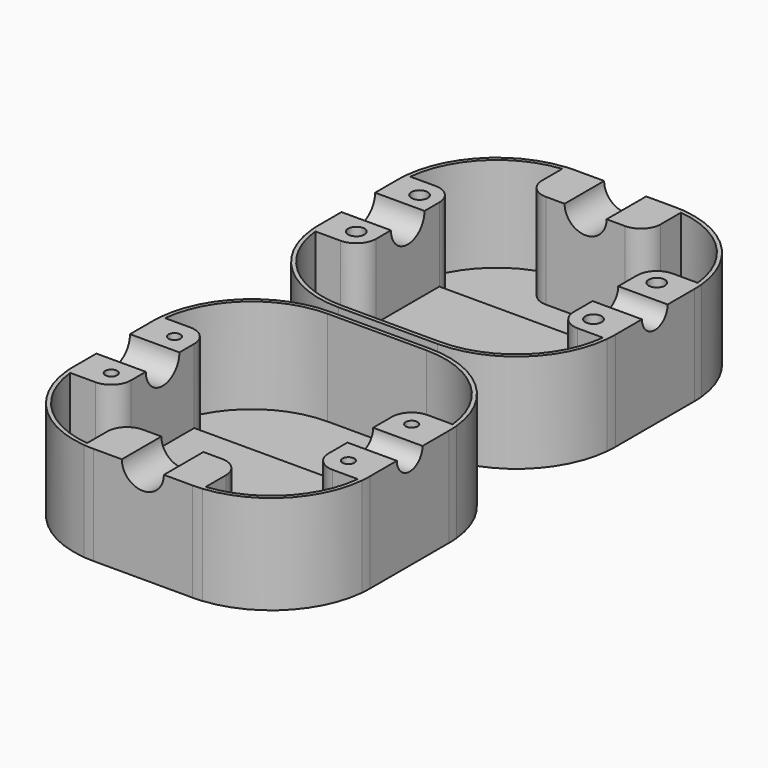
from build123d import *

# Parameters (mm, degrees)
F1_DEPTH        = 20
F2_T            = -0.8
F3_DEPTH        = 5
F4_DEPTH        = 20
F6_D            = 8.5
F6_DEPTH        = 12
F6_TIP          = 2.5536576309
F8_D            = 8.5
F8_DEPTH        = 12
F8_TIP          = 2.5536576309
F10_D           = 6.5
F10_DEPTH       = 12
F10_TIP         = 1.9527970118
F13_D           = 3.3
F13_CBORE_D     = 6.5
F13_CBORE_DEPTH = 6
F15_D           = 2.4
F15_DEPTH       = 17
F15_TIP         = 0.7210327428


# Not quite as in the source:
# - a feature names something its author has since deleted; it is built from what else it names


with BuildPart() as f1:
    # F0 (on Top) → F1 (new body)
    with BuildSketch(Plane.XY):
        with BuildLine():
            Line((-24, -12), (-29.8997487421, -12))
            ThreePointArc((-29.8997487421, -12), (-23.416407865, -24.8323969742), (-10, -30))
            Line((-10, -30), (0, -30))
            Line((0, -30), (10, -30))
            ThreePointArc((10, -30), (23.416407865, -24.8323969742), (29.8997487421, -12))
            Line((29.8997487421, -12), (24, -12))
            ThreePointArc((24, -12), (21.1715728753, -10.8284271247), (20, -8))
            Line((20, -8), (-20, -8))
            ThreePointArc((-20, -8), (-21.1715728753, -10.8284271247), (-24, -12))
        make_face()
        with BuildLine():
            Line((-24, 12), (-29.8997487421, 12))
            ThreePointArc((-29.8997487421, 12), (-29.9749214622, 11.0012555012), (-30, 10))
            Line((-30, 10), (-30, 0))
            Line((-30, 0), (-30, -10))
            ThreePointArc((-30, -10), (-29.9749214622, -11.0012555012), (-29.8997487421, -12))
            Line((-29.8997487421, -12), (-24, -12))
            ThreePointArc((-24, -12), (-21.1715728753, -10.8284271247), (-20, -8))
            Line((-20, -8), (-20, 0))
            Line((-20, 0), (-20, 8))
            ThreePointArc((-20, 8), (-21.1715728753, 10.8284271247), (-24, 12))
        make_face()
        with BuildLine():
            ThreePointArc((30, 10), (29.9749214622, 11.0012555012), (29.8997487421, 12))
            Line((29.8997487421, 12), (24, 12))
            ThreePointArc((24, 12), (21.1715728753, 10.8284271247), (20, 8))
            Line((20, 8), (20, 0))
            Line((20, 0), (20, -8))
            ThreePointArc((20, -8), (21.1715728753, -10.8284271247), (24, -12))
            Line((24, -12), (29.8997487421, -12))
            ThreePointArc((29.8997487421, -12), (29.9749214622, -11.0012555012), (30, -10))
            Line((30, -10), (30, 0))
            Line((30, 0), (30, 10))
        make_face()
        with BuildLine():
            Line((10, 30), (0, 30))
            Line((0, 30), (-10, 30))
            ThreePointArc((-10, 30), (-11.0012555012, 29.9749214622), (-12, 29.8997487421))
            Line((-12, 29.8997487421), (-12, 24))
            ThreePointArc((-12, 24), (-10.8284271247, 21.1715728753), (-8, 20))
            Line((-8, 20), (0, 20))
            Line((0, 20), (8, 20))
            ThreePointArc((8, 20), (10.8284271247, 21.1715728753), (12, 24))
            Line((12, 24), (12, 29.8997487421))
            ThreePointArc((12, 29.8997487421), (11.0012555012, 29.9749214622), (10, 30))
        make_face()
        with BuildLine():
            Line((-12, 24), (-12, 29.8997487421))
            ThreePointArc((-12, 29.8997487421), (-24.1421356237, 24.1421356237), (-29.8997487421, 12))
            Line((-29.8997487421, 12), (-24, 12))
            ThreePointArc((-24, 12), (-21.1715728753, 10.8284271247), (-20, 8))
            Line((-20, 8), (20, 8))
            ThreePointArc((20, 8), (21.1715728753, 10.8284271247), (24, 12))
            Line((24, 12), (29.8997487421, 12))
            ThreePointArc((29.8997487421, 12), (24.1421356237, 24.1421356237), (12, 29.8997487421))
            Line((12, 29.8997487421), (12, 24))
            ThreePointArc((12, 24), (10.8284271247, 21.1715728753), (8, 20))
            Line((8, 20), (0, 20))
            Line((0, 20), (-8, 20))
            ThreePointArc((-8, 20), (-10.8284271247, 21.1715728753), (-12, 24))
        make_face()
        Polygon((20, 8), (-20, 8), (-20, 0), (-20, -8), (20, -8), (20, 0), align=None)
    extrude(amount=F1_DEPTH)

    # F2
    f2_openings = [f1.faces().sort_by_distance(p)[0] for p in [
        (0, 0, 20),
    ]]
    offset(amount=F2_T, openings=f2_openings)

    # F0 (on Top) → F3 (join)
    with BuildSketch(Plane.XY):
        Polygon((20, 8), (-20, 8), (-20, 0), (-20, -8), (20, -8), (20, 0), align=None)
    extrude(amount=F3_DEPTH)

    # F0 (on Top) → F4 (join)
    with BuildSketch(Plane.XY):
        with BuildLine():
            ThreePointArc((30, 10), (29.9749214622, 11.0012555012), (29.8997487421, 12))
            Line((29.8997487421, 12), (24, 12))
            ThreePointArc((24, 12), (21.1715728753, 10.8284271247), (20, 8))
            Line((20, 8), (20, 0))
            Line((20, 0), (20, -8))
            ThreePointArc((20, -8), (21.1715728753, -10.8284271247), (24, -12))
            Line((24, -12), (29.8997487421, -12))
            ThreePointArc((29.8997487421, -12), (29.9749214622, -11.0012555012), (30, -10))
            Line((30, -10), (30, 0))
            Line((30, 0), (30, 10))
        make_face()
        with BuildLine():
            Line((10, 30), (0, 30))
            Line((0, 30), (-10, 30))
            ThreePointArc((-10, 30), (-11.0012555012, 29.9749214622), (-12, 29.8997487421))
            Line((-12, 29.8997487421), (-12, 24))
            ThreePointArc((-12, 24), (-10.8284271247, 21.1715728753), (-8, 20))
            Line((-8, 20), (0, 20))
            Line((0, 20), (8, 20))
            ThreePointArc((8, 20), (10.8284271247, 21.1715728753), (12, 24))
            Line((12, 24), (12, 29.8997487421))
            ThreePointArc((12, 29.8997487421), (11.0012555012, 29.9749214622), (10, 30))
        make_face()
        with BuildLine():
            Line((-24, 12), (-29.8997487421, 12))
            ThreePointArc((-29.8997487421, 12), (-29.9749214622, 11.0012555012), (-30, 10))
            Line((-30, 10), (-30, 0))
            Line((-30, 0), (-30, -10))
            ThreePointArc((-30, -10), (-29.9749214622, -11.0012555012), (-29.8997487421, -12))
            Line((-29.8997487421, -12), (-24, -12))
            ThreePointArc((-24, -12), (-21.1715728753, -10.8284271247), (-20, -8))
            Line((-20, -8), (-20, 0))
            Line((-20, 0), (-20, 8))
            ThreePointArc((-20, 8), (-21.1715728753, 10.8284271247), (-24, 12))
        make_face()
    extrude(amount=F4_DEPTH)

    # F6
    with Locations(Plane(origin=(-30, 0, 0), x_dir=(0, -1, 0), z_dir=(-1, 0, 0))):
        with Locations((0, 20)):
            Hole(F6_D / 2, depth=F6_DEPTH)
            with Locations((0, 0, -(F6_DEPTH + F6_TIP / 2))):  # 118° drill point
                Cone(0, F6_D / 2, F6_TIP, mode=Mode.SUBTRACT)

    # F8
    with Locations(Plane(origin=(0, 30, 0), x_dir=(-1, 0, 0), z_dir=(0, 1, 0))):
        with Locations((0, 20)):
            Hole(F8_D / 2, depth=F8_DEPTH)
            with Locations((0, 0, -(F8_DEPTH + F8_TIP / 2))):  # 118° drill point
                Cone(0, F8_D / 2, F8_TIP, mode=Mode.SUBTRACT)

    # F10
    with Locations(Plane.YZ.offset(30)):
        with Locations((0, 20)):
            Hole(F10_D / 2, depth=F10_DEPTH)
            with Locations((0, 0, -(F10_DEPTH + F10_TIP / 2))):  # 118° drill point
                Cone(0, F10_D / 2, F10_TIP, mode=Mode.SUBTRACT)


with BuildPart() as f12_1:
    # F12: instance of F1
    add(f1.part.mirror(Plane.XZ.offset(31)))

    # F15
    with Locations(Plane.XY.offset(20)):
        with Locations((-24, -54), (-24, -70), (24, -70), (24, -54)):
            Hole(F15_D / 2, depth=F15_DEPTH)
            with Locations((0, 0, -(F15_DEPTH + F15_TIP / 2))):  # 118° drill point
                Cone(0, F15_D / 2, F15_TIP, mode=Mode.SUBTRACT)


with BuildPart() as f1_1:
    add(f1.part)

    # F13 (through all)
    with Locations(Plane(origin=(0, 0, 0), x_dir=(1, 0, 0), z_dir=(0, 0, -1))):
        with Locations((-24, -8), (24, -8), (24, 8), (-24, 8)):
            CounterBoreHole(F13_D / 2, F13_CBORE_D / 2, F13_CBORE_DEPTH)


solid = Compound([f12_1.part, f1_1.part])
